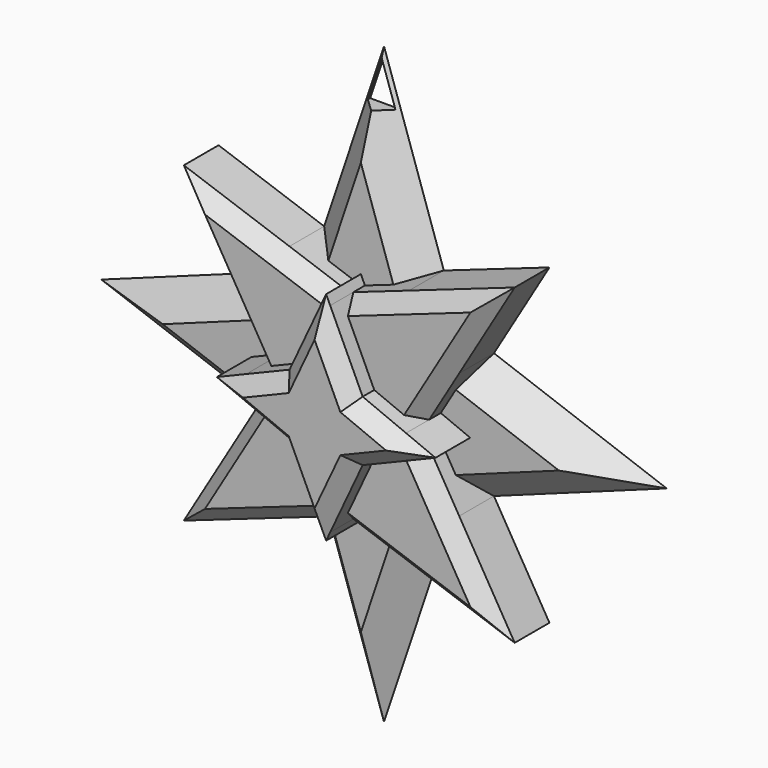
from build123d import *

# Parameters (mm, degrees)
F1_DEPTH       = 5.08
F2_DEPTH       = 10.16
F3_DEPTH       = 15.24
F5_DEPTH       = 25.4
F6_T1_DEPTH    = 43.0847621983
F6_T3_DEPTH    = 42.4996652057
F6_2_T1_DEPTH  = 42.4996652057
F6_2_T3_DEPTH  = 43.0847621983
F6_3_T1_DEPTH  = 43.0847621983
F6_3_T3_DEPTH  = 42.4996652057
F6_4_T1_DEPTH  = 42.4996652057
F6_4_T3_DEPTH  = 43.0847621983
F6_5_T4_DEPTH  = 28.2434080268
F6_5_T9_DEPTH  = 28.2434080268
F6_5_T14_DEPTH = 26.8952157279
F6_5_T19_DEPTH = 26.8952157279
F6_5_T24_DEPTH = 28.2434080268
F6_5_T29_DEPTH = 28.2434080268
F6_5_T34_DEPTH = 26.8952157279
F6_5_T39_DEPTH = 26.8952157279
F6_5_T45_DEPTH = 28.2434080268
F6_5_T49_DEPTH = 26.8952157279
F6_5_T56_DEPTH = 26.8952157279
F6_5_T60_DEPTH = 28.2434080268
F6_5_T67_DEPTH = 28.2434080268
F6_5_T71_DEPTH = 26.8952157279
F6_5_T78_DEPTH = 26.8952157279
F6_5_T82_DEPTH = 28.2434080268
F7_C1_SIZE     = 5.0799
F7_C2_SIZE     = 5.0799
F7_2_T1_DEPTH  = 59.1132304118
F7_2_T3_DEPTH  = 59.1132304118
F7_3_C1_SIZE   = 5.0799
F7_3_C2_SIZE   = 5.0799
F7_4_C1_SIZE   = 5.0799
F7_4_C2_SIZE   = 5.0799


# Not quite as in the source:
# - a fillet or chamfer that OpenCascade refuses, or shapes differently, is made with other operations: its cross-section is extruded or revolved along the edge and cut away or added
# - a fillet or chamfer is up to 0.001 mm smaller than in the source, because OpenCascade refuses the exact size


with BuildPart() as f1:
    # F0 (on Front) → F1 (new body)
    with BuildSketch(Plane.XZ):
        Polygon((-19.1932707477, 0), (-49.6243569425, 0), (-19.302516341, -11.0362474271), (-14.0268384734, -2.1400063171), align=None)
        Polygon((-19.302516341, 11.0362474271), (-49.6243569425, 0), (-19.1932707477, 0), (-14.0268384734, 2.1400063171), align=None)
    extrude(amount=F1_DEPTH)

    # F7: chamfer of 5.08 on 2 edges, made by hand

    # F7_c1 (size 5.08 in the source; OpenCascade refuses exactly that, so slightly less here)
    f7_c1_edges = [f1.edges().sort_by_distance(p)[0] for p in [
        (-34.4634366418, -5.08, 5.5181237136),
    ]]
    chamfer(f7_c1_edges, length=F7_C1_SIZE)

    # F7_c2 (size 5.08 in the source; OpenCascade refuses exactly that, so slightly less here)
    f7_c2_edges = [f1.edges().sort_by_distance(p)[0] for p in [
        (-30.7502781487, -5.08, -6.8696028802),
    ]]
    chamfer(f7_c2_edges, length=F7_C2_SIZE)


with BuildPart() as f1b:
    # F0 (on Front) → F1, piece 2 (new body)
    with BuildSketch(Plane.XZ):
        Polygon((10.5027486839, 20.9549840158), (0, 52.2231460967), (0, 19.05), (0.7131063295, 17.5207385413), align=None)
        Polygon((0, 52.2231460967), (-10.5027486839, 20.9549840158), (-0.7131063295, 17.5207385413), (0, 19.05), align=None)
    extrude(amount=F1_DEPTH)

    # F4 (on face) → F5 (cut)
    with BuildSketch(Plane.XZ.offset(5.08)):
        Polygon((2.4262880633, 43.3883815264), (0, 50.611782819), (-2.4262880633, 43.3883815264), align=None)
    extrude(amount=-F5_DEPTH, mode=Mode.SUBTRACT)

    # F7#2: chamfer of 5.08 on 2 edges, made by hand

    # F7_2_s2 → F7_2_t1 (cut)
    with BuildSketch(Plane(origin=(-1.1004277598, 0, 3.2761284296), x_dir=(0, 1, 0), z_dir=(-0.318410507, 0, 0.9479529255))):
        Polygon((-5.08, -11.5483984258), (0, -16.6283984258), (-5.08, -16.6283984258), align=None)
    extrude(amount=F7_2_T1_DEPTH, mode=Mode.SUBTRACT)

    # F7_2_s4 → F7_2_t3 (cut)
    with BuildSketch(Plane(origin=(19.9227014256, 0, 59.3126881363), x_dir=(0, 1, 0), z_dir=(-0.318410507, 0, -0.9479529255))):
        Polygon((-5.08, -11.5483984258), (0, -16.6283984258), (-5.08, -16.6283984258), align=None)
    extrude(amount=F7_2_T3_DEPTH, mode=Mode.SUBTRACT)


with BuildPart() as f1c:
    # F0 (on Front) → F1, piece 3 (new body)
    with BuildSketch(Plane.XZ):
        Polygon((49.6243569425, 0), (19.302516341, 11.0362474271), (14.0268384734, 2.1400063171), (19.1932707477, 0), align=None)
        Polygon((14.0268384734, -2.1400063171), (19.302516341, -11.0362474271), (49.6243569425, 0), (19.1932707477, 0), align=None)
    extrude(amount=F1_DEPTH)

    # F7#3: chamfer of 5.08 on 2 edges, made by hand

    # F7_3_c1 (size 5.08 in the source; OpenCascade refuses exactly that, so slightly less here)
    f7_3_c1_edges = [f1c.edges().sort_by_distance(p)[0] for p in [
        (34.4634366418, -5.08, -5.5181237136),
    ]]
    chamfer(f7_3_c1_edges, length=F7_3_C1_SIZE)

    # F7_3_c2 (size 5.08 in the source; OpenCascade refuses exactly that, so slightly less here)
    f7_3_c2_edges = [f1c.edges().sort_by_distance(p)[0] for p in [
        (30.7502781487, -5.08, 6.8696028802),
    ]]
    chamfer(f7_3_c2_edges, length=F7_3_C2_SIZE)


with BuildPart() as f1d:
    # F0 (on Front) → F1, piece 4 (new body)
    with BuildSketch(Plane.XZ):
        Polygon((0, -19.05), (0, -52.2231460967), (10.5027486839, -20.9549840158), (0.7131063295, -17.5207385413), align=None)
        Polygon((-0.7131063295, -17.5207385413), (-10.5027486839, -20.9549840158), (0, -52.2231460967), (0, -19.05), align=None)
    extrude(amount=F1_DEPTH)

    # F7#4: chamfer of 5.08 on 2 edges, made by hand

    # F7_4_c1 (size 5.08 in the source; OpenCascade refuses exactly that, so slightly less here)
    f7_4_c1_edges = [f1d.edges().sort_by_distance(p)[0] for p in [
        (-5.251374342, -5.08, -36.5890650563),
    ]]
    chamfer(f7_4_c1_edges, length=F7_4_C1_SIZE)

    # F7_4_c2 (size 5.08 in the source; OpenCascade refuses exactly that, so slightly less here)
    f7_4_c2_edges = [f1d.edges().sort_by_distance(p)[0] for p in [
        (6.591076943, -5.08, -32.6005817239),
    ]]
    chamfer(f7_4_c2_edges, length=F7_4_C2_SIZE)


with BuildPart() as f2:
    # F0 (on Front) → F2 (new body)
    with BuildSketch(Plane.XZ):
        Polygon((-29.0412037669, 27.4583477923), (-19.302516341, 11.0362474271), (-14.0268384734, 2.1400063171), (-6.4150318198, 5.2929198672), (-0.7131063295, 17.5207385413), (-10.5027486839, 20.9549840158), align=None)
    extrude(amount=F2_DEPTH)

    # F6: chamfer of 2.54 on 2 edges, made by hand

    # F6_s2 → F6_t1 (cut)
    with BuildSketch(Plane(origin=(-40.5997078736, 0, 14.2425390001), x_dir=(0, 1, 0), z_dir=(0.9436215642, 0, -0.3310261978))):
        Polygon((-7.62, 16.296889831), (-10.16, 13.756889831), (-10.16, 16.296889831), align=None)
    extrude(amount=F6_T1_DEPTH, mode=Mode.SUBTRACT)

    # F6_s4 → F6_t3 (cut)
    with BuildSketch(Plane(origin=(-1.256506008, 0, 2.1188140527), x_dir=(0, 1, 0), z_dir=(-0.5100765172, 0, 0.860129029))):
        Polygon((-10.16, 8.4333239875), (-7.62, 10.9733239875), (-10.16, 10.9733239875), align=None)
    extrude(amount=F6_T3_DEPTH, mode=Mode.SUBTRACT)


with BuildPart() as f2b:
    # F0 (on Front) → F2, piece 2 (new body)
    with BuildSketch(Plane.XZ):
        Polygon((-14.0268384734, -2.1400063171), (-19.302516341, -11.0362474271), (-29.0412037669, -27.4583477923), (-10.5027486839, -20.9549840158), (-0.7131063295, -17.5207385413), (-6.4150318198, -5.2929198672), align=None)
    extrude(amount=F2_DEPTH)

    # F6#2: chamfer of 2.54 on 2 edges, made by hand

    # F6_2_s2 → F6_2_t1 (cut)
    with BuildSketch(Plane(origin=(-22.934587219, 0, -38.6740098203), x_dir=(0, 1, 0), z_dir=(0.5100765172, 0, 0.860129029))):
        Polygon((-10.16, 8.4333239875), (-7.62, 10.9733239875), (-10.16, 10.9733239875), align=None)
    extrude(amount=F6_2_T1_DEPTH, mode=Mode.SUBTRACT)

    # F6_2_s4 → F6_2_t3 (cut)
    with BuildSketch(Plane(origin=(0.056002824, 0, 0.0196460134), x_dir=(0, 1, 0), z_dir=(-0.9436215642, 0, -0.3310261978))):
        Polygon((-10.16, 13.756889831), (-7.62, 16.296889831), (-10.16, 16.296889831), align=None)
    extrude(amount=F6_2_T3_DEPTH, mode=Mode.SUBTRACT)


with BuildPart() as f2c:
    # F0 (on Front) → F2, piece 3 (new body)
    with BuildSketch(Plane.XZ):
        Polygon((0.7131063295, -17.5207385413), (10.5027486839, -20.9549840158), (29.0412037669, -27.4583477923), (19.302516341, -11.0362474271), (14.0268384734, -2.1400063171), (6.4150318198, -5.2929198672), align=None)
    extrude(amount=F2_DEPTH)

    # F6#3: chamfer of 2.54 on 2 edges, made by hand

    # F6_3_s2 → F6_3_t1 (cut)
    with BuildSketch(Plane(origin=(40.5997078736, 0, -14.2425390001), x_dir=(0, 1, 0), z_dir=(-0.9436215642, 0, 0.3310261978))):
        Polygon((-10.16, 13.756889831), (-7.62, 16.296889831), (-10.16, 16.296889831), align=None)
    extrude(amount=F6_3_T1_DEPTH, mode=Mode.SUBTRACT)

    # F6_3_s4 → F6_3_t3 (cut)
    with BuildSketch(Plane(origin=(1.256506008, 0, -2.1188140527), x_dir=(0, 1, 0), z_dir=(0.5100765172, 0, -0.860129029))):
        Polygon((-10.16, 8.4333239875), (-7.62, 10.9733239875), (-10.16, 10.9733239875), align=None)
    extrude(amount=F6_3_T3_DEPTH, mode=Mode.SUBTRACT)


with BuildPart() as f2d:
    # F0 (on Front) → F2, piece 4 (new body)
    with BuildSketch(Plane.XZ):
        Polygon((29.0412037669, 27.4583477923), (10.5027486839, 20.9549840158), (0.7131063295, 17.5207385413), (6.4150318198, 5.2929198672), (14.0268384734, 2.1400063171), (19.302516341, 11.0362474271), align=None)
    extrude(amount=F2_DEPTH)

    # F6#4: chamfer of 2.54 on 2 edges, made by hand

    # F6_4_s2 → F6_4_t1 (cut)
    with BuildSketch(Plane(origin=(22.934587219, 0, 38.6740098203), x_dir=(0, 1, 0), z_dir=(-0.5100765172, 0, -0.860129029))):
        Polygon((-7.62, 10.9733239875), (-10.16, 8.4333239875), (-10.16, 10.9733239875), align=None)
    extrude(amount=F6_4_T1_DEPTH, mode=Mode.SUBTRACT)

    # F6_4_s4 → F6_4_t3 (cut)
    with BuildSketch(Plane(origin=(-0.056002824, 0, -0.0196460134), x_dir=(0, 1, 0), z_dir=(0.9436215642, 0, 0.3310261978))):
        Polygon((-10.16, 13.756889831), (-7.62, 16.296889831), (-10.16, 16.296889831), align=None)
    extrude(amount=F6_4_T3_DEPTH, mode=Mode.SUBTRACT)


with BuildPart() as f3:
    # F0 (on Front) → F3 (new body)
    with BuildSketch(Plane.XZ):
        Polygon((-14.0268384734, 2.1400063171), (-19.1932707477, 0), (-14.0268384734, -2.1400063171), (-6.4150318198, -5.2929198672), (-0.7131063295, -17.5207385413), (0, -19.05), (0.7131063295, -17.5207385413), (6.4150318198, -5.2929198672), (14.0268384734, -2.1400063171), (19.1932707477, 0), (14.0268384734, 2.1400063171), (6.4150318198, 5.2929198672), (0.7131063295, 17.5207385413), (0, 19.05), (-0.7131063295, 17.5207385413), (-6.4150318198, 5.2929198672), align=None)
    extrude(amount=F3_DEPTH)

    # F6#5: chamfer of 2.54 on 8 edges, made by hand


with BuildPart() as f6_5_tool2:
    # F6_5_s3 → F6_5_t4 (new body)
    with BuildSketch(Plane(origin=(10.0571474138, 0, -21.5676222294), x_dir=(0, 1, 0), z_dir=(-0.4226182617, 0, 0.906307787))):
        Polygon((-12.7, 8.0508778862), (-15.24, 5.5108778862), (-15.24, 8.0508778862), align=None)
    extrude(amount=F6_5_T4_DEPTH)

    split(bisect_by=Plane(origin=(-2.8107894244, 0, -6.7858459494), x_dir=(0, 1, 0), z_dir=(-0.3826834324, 0, -0.9238795325)), keep=Keep.TOP)


with BuildPart() as f3_1:
    add(f3.part)

    # F6_5_t1: cut F6_5_tool2
    add(f6_5_tool2.part, mode=Mode.SUBTRACT)


with BuildPart() as f6_5_tool7:
    # F6_5_s8 → F6_5_t9 (new body)
    with BuildSketch(Plane(origin=(1.8790325922, 0, 4.0295983977), x_dir=(0, 1, 0), z_dir=(-0.4226182617, 0, -0.906307787))):
        Polygon((-12.7, 8.0508778862), (-15.24, 5.5108778862), (-15.24, 8.0508778862), align=None)
    extrude(amount=F6_5_T9_DEPTH)

    split(bisect_by=Plane(origin=(2.8107894244, 0, -6.7858459494), x_dir=(0, 1, 0), z_dir=(0.3826834324, 0, -0.9238795325)), keep=Keep.TOP)


with BuildPart() as f3_2:
    add(f3_1.part)

    # F6_5_t6: cut F6_5_tool7
    add(f6_5_tool7.part, mode=Mode.SUBTRACT)


with BuildPart() as f6_5_tool12:
    # F6_5_s13 → F6_5_t14 (new body)
    with BuildSketch(Plane(origin=(22.417331526, 0, 9.2855627503), x_dir=(0, 1, 0), z_dir=(-0.9238795325, 0, -0.3826834324))):
        Polygon((-12.7, 7.344946728), (-15.24, 4.804946728), (-15.24, 7.344946728), align=None)
    extrude(amount=F6_5_T14_DEPTH)

    split(bisect_by=Plane(origin=(7.2965733207, 0, -3.4024480177), x_dir=(0, 1, 0), z_dir=(0.906307787, 0, -0.4226182617)), keep=Keep.TOP)


with BuildPart() as f3_3:
    add(f3_2.part)

    # F6_5_t11: cut F6_5_tool12
    add(f6_5_tool12.part, mode=Mode.SUBTRACT)


with BuildPart() as f6_5_tool17:
    # F6_5_s18 → F6_5_t19 (new body)
    with BuildSketch(Plane(origin=(-2.4306078074, 0, 1.0067907186), x_dir=(0, 1, 0), z_dir=(0.9238795325, 0, -0.3826834324))):
        Polygon((-12.7, 7.344946728), (-15.24, 4.804946728), (-15.24, 7.344946728), align=None)
    extrude(amount=F6_5_T19_DEPTH)

    split(bisect_by=Plane(origin=(7.2965733207, 0, 3.4024480177), x_dir=(0, 1, 0), z_dir=(0.906307787, 0, 0.4226182617)), keep=Keep.TOP)


with BuildPart() as f3_4:
    add(f3_3.part)

    # F6_5_t16: cut F6_5_tool17
    add(f6_5_tool17.part, mode=Mode.SUBTRACT)


with BuildPart() as f6_5_tool22:
    # F6_5_s23 → F6_5_t24 (new body)
    with BuildSketch(Plane(origin=(-10.0571474138, 0, 21.5676222294), x_dir=(0, 1, 0), z_dir=(0.4226182617, 0, -0.906307787))):
        Polygon((-12.7, 8.0508778862), (-15.24, 5.5108778862), (-15.24, 8.0508778862), align=None)
    extrude(amount=F6_5_T24_DEPTH)

    split(bisect_by=Plane(origin=(2.8107894244, 0, 6.7858459494), x_dir=(0, 1, 0), z_dir=(0.3826834324, 0, 0.9238795325)), keep=Keep.TOP)


with BuildPart() as f3_5:
    add(f3_4.part)

    # F6_5_t21: cut F6_5_tool22
    add(f6_5_tool22.part, mode=Mode.SUBTRACT)


with BuildPart() as f6_5_tool27:
    # F6_5_s28 → F6_5_t29 (new body)
    with BuildSketch(Plane(origin=(-1.8790325922, 0, -4.0295983977), x_dir=(0, 1, 0), z_dir=(0.4226182617, 0, 0.906307787))):
        Polygon((-15.24, 5.5108778862), (-12.7, 8.0508778862), (-15.24, 8.0508778862), align=None)
    extrude(amount=F6_5_T29_DEPTH)

    split(bisect_by=Plane(origin=(-2.8107894244, 0, 6.7858459494), x_dir=(0, 1, 0), z_dir=(-0.3826834324, 0, 0.9238795325)), keep=Keep.TOP)


with BuildPart() as f3_6:
    add(f3_5.part)

    # F6_5_t26: cut F6_5_tool27
    add(f6_5_tool27.part, mode=Mode.SUBTRACT)


with BuildPart() as f6_5_tool32:
    # F6_5_s33 → F6_5_t34 (new body)
    with BuildSketch(Plane(origin=(-22.417331526, 0, -9.2855627503), x_dir=(0, 1, 0), z_dir=(0.9238795325, 0, 0.3826834324))):
        Polygon((-12.7, 7.344946728), (-15.24, 4.804946728), (-15.24, 7.344946728), align=None)
    extrude(amount=F6_5_T34_DEPTH)

    split(bisect_by=Plane(origin=(-7.2965733207, 0, 3.4024480177), x_dir=(0, 1, 0), z_dir=(-0.906307787, 0, 0.4226182617)), keep=Keep.TOP)


with BuildPart() as f3_7:
    add(f3_6.part)

    # F6_5_t31: cut F6_5_tool32
    add(f6_5_tool32.part, mode=Mode.SUBTRACT)


with BuildPart() as f6_5_tool37:
    # F6_5_s38 → F6_5_t39 (new body)
    with BuildSketch(Plane(origin=(2.4306078074, 0, -1.0067907186), x_dir=(0, 1, 0), z_dir=(-0.9238795325, 0, 0.3826834324))):
        Polygon((-12.7, 7.344946728), (-15.24, 4.804946728), (-15.24, 7.344946728), align=None)
    extrude(amount=F6_5_T39_DEPTH)

    split(bisect_by=Plane(origin=(-7.2965733207, 0, -3.4024480177), x_dir=(0, 1, 0), z_dir=(-0.906307787, 0, -0.4226182617)), keep=Keep.TOP)


with BuildPart() as f3_8:
    add(f3_7.part)

    # F6_5_t36: cut F6_5_tool37
    add(f6_5_tool37.part, mode=Mode.SUBTRACT)


with BuildPart() as f6_5_tool43:
    # F6_5_s44 → F6_5_t45 (new body)
    with BuildSketch(Plane(origin=(10.0571474138, 0, -21.5676222294), x_dir=(0, 1, 0), z_dir=(-0.4226182617, 0, 0.906307787))):
        Polygon((-12.7, 8.0508778862), (-15.24, 5.5108778862), (-15.24, 8.0508778862), align=None)
    extrude(amount=F6_5_T45_DEPTH)

    split(bisect_by=Plane(origin=(-2.8107894244, 0, -6.7858459494), x_dir=(0, 1, 0), z_dir=(0.3826834324, 0, 0.9238795325)), keep=Keep.TOP)


with BuildPart() as f6_5_tool47:
    # F6_5_s48 → F6_5_t49 (new body)
    with BuildSketch(Plane(origin=(2.4306078074, 0, -1.0067907186), x_dir=(0, 1, 0), z_dir=(-0.9238795325, 0, 0.3826834324))):
        Polygon((-12.7, 7.344946728), (-15.24, 4.804946728), (-15.24, 7.344946728), align=None)
    extrude(amount=F6_5_T49_DEPTH)

    split(bisect_by=Plane(origin=(-7.2965733207, 0, -3.4024480177), x_dir=(0, 1, 0), z_dir=(0.906307787, 0, 0.4226182617)), keep=Keep.TOP)


with BuildPart() as f6_5_tool43_1:
    add(f6_5_tool43.part)

    # F6_5_t51: intersect F6_5_tool47
    add(f6_5_tool47.part, mode=Mode.INTERSECT)


with BuildPart() as f3_9:
    add(f3_8.part)

    # F6_5_t41: cut F6_5_tool43
    add(f6_5_tool43_1.part, mode=Mode.SUBTRACT)


with BuildPart() as f6_5_tool54:
    # F6_5_s55 → F6_5_t56 (new body)
    with BuildSketch(Plane(origin=(22.417331526, 0, 9.2855627503), x_dir=(0, 1, 0), z_dir=(-0.9238795325, 0, -0.3826834324))):
        Polygon((-12.7, 7.344946728), (-15.24, 4.804946728), (-15.24, 7.344946728), align=None)
    extrude(amount=F6_5_T56_DEPTH)

    split(bisect_by=Plane(origin=(7.2965733207, 0, -3.4024480177), x_dir=(0, 1, 0), z_dir=(-0.906307787, 0, 0.4226182617)), keep=Keep.TOP)


with BuildPart() as f6_5_tool58:
    # F6_5_s59 → F6_5_t60 (new body)
    with BuildSketch(Plane(origin=(1.8790325922, 0, 4.0295983977), x_dir=(0, 1, 0), z_dir=(-0.4226182617, 0, -0.906307787))):
        Polygon((-12.7, 8.0508778862), (-15.24, 5.5108778862), (-15.24, 8.0508778862), align=None)
    extrude(amount=F6_5_T60_DEPTH)

    split(bisect_by=Plane(origin=(2.8107894244, 0, -6.7858459494), x_dir=(0, 1, 0), z_dir=(-0.3826834324, 0, 0.9238795325)), keep=Keep.TOP)


with BuildPart() as f6_5_tool54_1:
    add(f6_5_tool54.part)

    # F6_5_t62: intersect F6_5_tool58
    add(f6_5_tool58.part, mode=Mode.INTERSECT)


with BuildPart() as f3_10:
    add(f3_9.part)

    # F6_5_t52: cut F6_5_tool54
    add(f6_5_tool54_1.part, mode=Mode.SUBTRACT)


with BuildPart() as f6_5_tool65:
    # F6_5_s66 → F6_5_t67 (new body)
    with BuildSketch(Plane(origin=(-10.0571474138, 0, 21.5676222294), x_dir=(0, 1, 0), z_dir=(0.4226182617, 0, -0.906307787))):
        Polygon((-12.7, 8.0508778862), (-15.24, 5.5108778862), (-15.24, 8.0508778862), align=None)
    extrude(amount=F6_5_T67_DEPTH)

    split(bisect_by=Plane(origin=(2.8107894244, 0, 6.7858459494), x_dir=(0, 1, 0), z_dir=(-0.3826834324, 0, -0.9238795325)), keep=Keep.TOP)


with BuildPart() as f6_5_tool69:
    # F6_5_s70 → F6_5_t71 (new body)
    with BuildSketch(Plane(origin=(-2.4306078074, 0, 1.0067907186), x_dir=(0, 1, 0), z_dir=(0.9238795325, 0, -0.3826834324))):
        Polygon((-12.7, 7.344946728), (-15.24, 4.804946728), (-15.24, 7.344946728), align=None)
    extrude(amount=F6_5_T71_DEPTH)

    split(bisect_by=Plane(origin=(7.2965733207, 0, 3.4024480177), x_dir=(0, 1, 0), z_dir=(-0.906307787, 0, -0.4226182617)), keep=Keep.TOP)


with BuildPart() as f6_5_tool65_1:
    add(f6_5_tool65.part)

    # F6_5_t73: intersect F6_5_tool69
    add(f6_5_tool69.part, mode=Mode.INTERSECT)


with BuildPart() as f3_11:
    add(f3_10.part)

    # F6_5_t63: cut F6_5_tool65
    add(f6_5_tool65_1.part, mode=Mode.SUBTRACT)


with BuildPart() as f6_5_tool76:
    # F6_5_s77 → F6_5_t78 (new body)
    with BuildSketch(Plane(origin=(-22.417331526, 0, -9.2855627503), x_dir=(0, 1, 0), z_dir=(0.9238795325, 0, 0.3826834324))):
        Polygon((-12.7, 7.344946728), (-15.24, 4.804946728), (-15.24, 7.344946728), align=None)
    extrude(amount=F6_5_T78_DEPTH)

    split(bisect_by=Plane(origin=(-7.2965733207, 0, 3.4024480177), x_dir=(0, 1, 0), z_dir=(0.906307787, 0, -0.4226182617)), keep=Keep.TOP)


with BuildPart() as f6_5_tool80:
    # F6_5_s81 → F6_5_t82 (new body)
    with BuildSketch(Plane(origin=(-1.8790325922, 0, -4.0295983977), x_dir=(0, 1, 0), z_dir=(0.4226182617, 0, 0.906307787))):
        Polygon((-15.24, 5.5108778862), (-12.7, 8.0508778862), (-15.24, 8.0508778862), align=None)
    extrude(amount=F6_5_T82_DEPTH)

    split(bisect_by=Plane(origin=(-2.8107894244, 0, 6.7858459494), x_dir=(0, 1, 0), z_dir=(0.3826834324, 0, -0.9238795325)), keep=Keep.TOP)


with BuildPart() as f6_5_tool76_1:
    add(f6_5_tool76.part)

    # F6_5_t84: intersect F6_5_tool80
    add(f6_5_tool80.part, mode=Mode.INTERSECT)


with BuildPart() as f3_12:
    add(f3_11.part)

    # F6_5_t74: cut F6_5_tool76
    add(f6_5_tool76_1.part, mode=Mode.SUBTRACT)


solid = Compound([f1.part, f1b.part, f1c.part, f1d.part, f2.part, f2b.part, f2c.part, f2d.part, f3_12.part])
